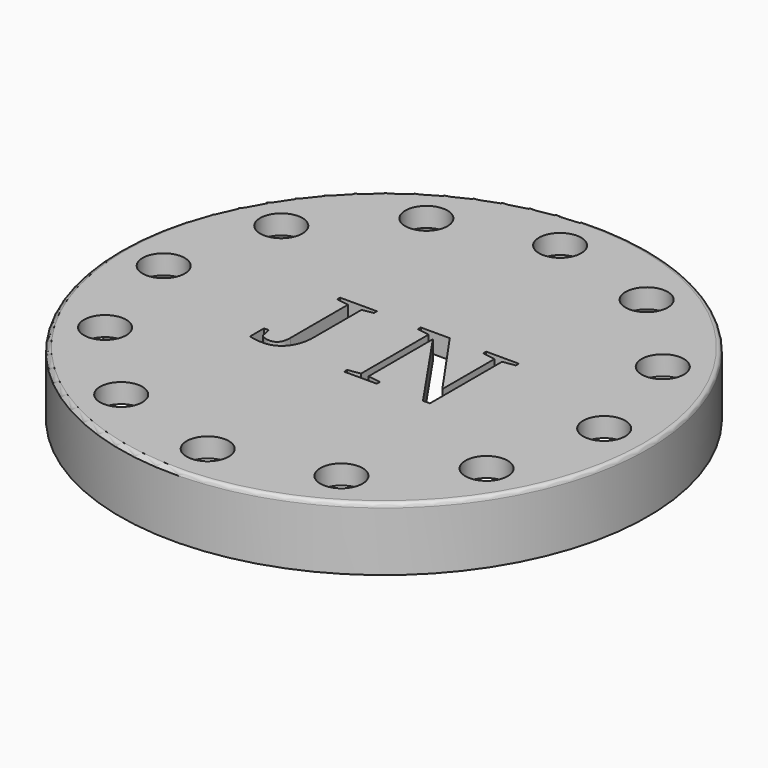
from build123d import *

# Parameters (mm, degrees)
F2_R         = 1
F3_R         = 0.5
F4_R         = 2.5
F5_DEPTH     = 7.501
F6_TEXT_SIZE = 17.3165087795
F7_DEPTH     = 7.501


# Not quite as in the source:
# - Text() gives the source's letters only with a copy of the font that has no kerning and outlines rounded to 1/6400 em; it was checked with that copy


with BuildPart() as f1:
    # F0 (on Front) → F1 (revolve)
    with BuildSketch(Plane.XZ):
        Polygon((0, 8.5062808216), (0, 10.8062808216), (-31.25, 10.8062808216), (-31.25, 3.3062808216), (-29.25, 3.3062808216), (-29.25, 4.7062808216), (-29.75, 4.7062808216), (-29.75, 8.5062808216), align=None)
    revolve(axis=Axis((0, 0, 9.6562808216), (0, 0, 1)))

    # F2
    f2_edges = [f1.edges().sort_by_distance(p)[0] for p in [
        (29.75, 0, 8.506281),
    ]]
    fillet(f2_edges, radius=F2_R)

    # F3
    f3_edges = [f1.edges().sort_by_distance(p)[0] for p in [
        (31.25, 0, 10.806281),
    ]]
    fillet(f3_edges, radius=F3_R)

    # F4 (on face) → F5 (cut, through all)
    with BuildSketch(Plane.XY.offset(10.8062808216)):
        with Locations((-22.5830574571, 13.038334302)):
            Circle(F4_R)
        with Locations((-26.076668604, 0)):
            Circle(F4_R)
        with Locations((-22.5830574571, -13.038334302)):
            Circle(F4_R)
        with Locations((-13.038334302, -22.5830574571)):
            Circle(F4_R)
        with Locations((0, -26.076668604)):
            Circle(F4_R)
        with Locations((13.038334302, -22.5830574571)):
            Circle(F4_R)
        with Locations((22.5830574571, -13.038334302)):
            Circle(F4_R)
        with Locations((26.076668604, 0)):
            Circle(F4_R)
        with Locations((22.5830574571, 13.038334302)):
            Circle(F4_R)
        with Locations((13.038334302, 22.5830574571)):
            Circle(F4_R)
        with Locations((0, 26.076668604)):
            Circle(F4_R)
        with Locations((-13.038334302, 22.5830574571)):
            Circle(F4_R)
    extrude(amount=-F5_DEPTH, mode=Mode.SUBTRACT)

    # F6 (on face) → F7 (cut, through all)
    with BuildSketch(Plane.XY.offset(10.8062808216)):
        with Locations((-11.3680549393, -6.1346981674)):
            Text('J N', F6_TEXT_SIZE, font='Tinos', text_align=(TextAlign.LEFT, TextAlign.BOTTOM))
    extrude(amount=-F7_DEPTH, mode=Mode.SUBTRACT)


solid = f1.part
